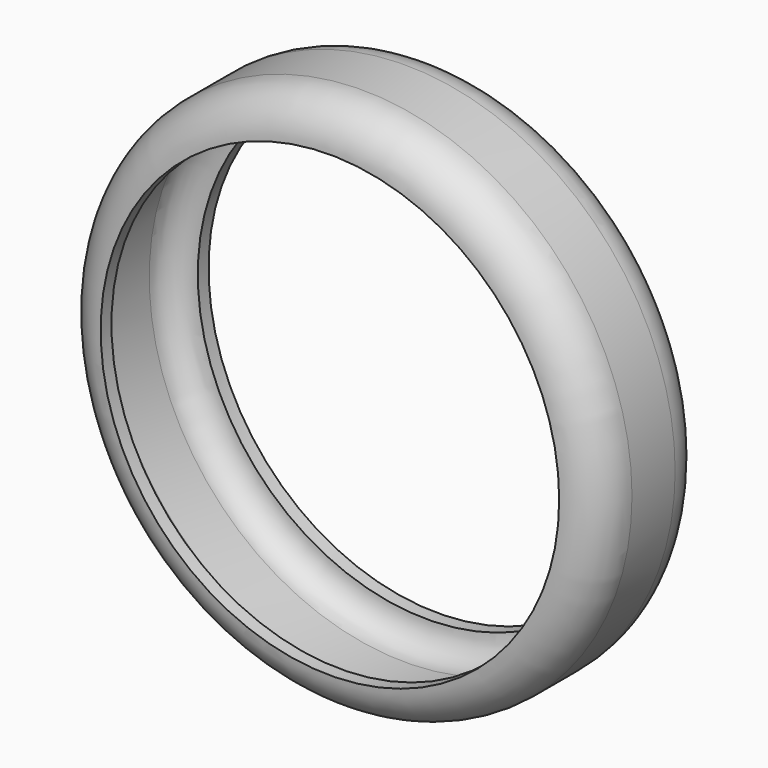
from build123d import *

# Parameters (mm, degrees)
F0_R     = 50.8
F1_DEPTH = 25.4
F2_R     = 7.62
F3_T     = -2.54


# Not quite as in the source:
# - a shell that OpenCascade refuses in one call is made with other operations: the cavity is built on its own and cut out


with BuildPart() as f1:
    # F0 (on Front) → F1 (new body)
    with BuildSketch(Plane.XZ):
        Circle(F0_R)
    extrude(amount=F1_DEPTH)

    # F2
    f2_edges = [f1.edges().sort_by_distance(p)[0] for p in [
        (-50.8, -25.4, 0),
        (-50.8, 0, 0),
    ]]
    fillet(f2_edges, radius=F2_R)

    # F3: a shell. OpenCascade refuses it in one call, so the cavity is built on its own and cut out:
    # the body offset inwards by the wall thickness, plus a prism from it out through each open face.
    f3_core = offset(f1.part, amount=F3_T, mode=Mode.PRIVATE)
    f3_exits = [f3_core.faces().sort_by_distance(p)[0] for p in [
        (0, -22.86, 0),
        (0, -2.54, 0),
    ]]
    add(f3_core, mode=Mode.SUBTRACT)
    extrude(f3_exits, amount=-F3_T, mode=Mode.SUBTRACT)


solid = f1.part
